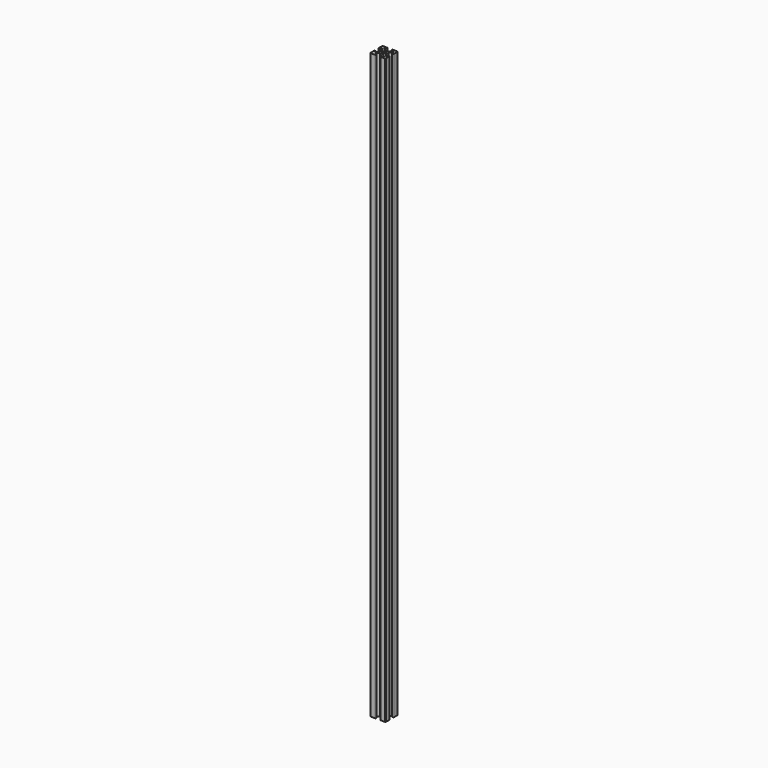
from build123d import *

# Parameters (mm, degrees)
F2_DEPTH = 760
F4_R     = 0.5
F5_R     = 1
F6_COUNT = 4


with BuildPart() as f2:
    # F1 (on Top) → F2 (new body)
    with BuildSketch(Plane.XY):
        with BuildLine():
            Line((3.0000000262, 10), (3.0000000262, 8))
            Line((3.0000000262, 8), (6.0000000262, 8))
            Line((6.0000000262, 8), (6.0000000262, 7.6925075952))
            Line((6.0000000262, 7.6925075952), (2.290812958, 4.0206899498))
            Line((2.290812958, 4.0206899498), (0.2126651618, 4))
            Line((0.2126651618, 4), (-0.0373348382, 3.75))
            Line((-0.0373348382, 3.75), (-0.0209097774, 2.1002278027))
            ThreePointArc((-0.0209097774, 2.1002278027), (1.4776309645, 1.4925138011), (2.1, 0))
            Line((2.1, 0), (3.7501858474, 0))
            Line((3.7501858474, 0), (4.0001858474, 0.25))
            Line((4.0001858474, 0.25), (3.9833205532, 2.3281823546))
            Line((3.9833205532, 2.3281823546), (7.6925076214, 6))
            Line((7.6925076214, 6), (8.0000000262, 6))
            Line((8.0000000262, 6), (8.0000000262, 3))
            Line((8.0000000262, 3), (10.0000000262, 3))
            Line((10.0000000262, 3), (10.0000000262, 10))
            Line((10.0000000262, 10), (3.0000000262, 10))
        make_face()
    extrude(amount=F2_DEPTH)

    # F4
    f4_edges = [f2.edges().sort_by_distance(p)[0] for p in [
        (3, 10, 380),
        (10, 3, 380),
        (8, 3, 380),
        (3, 8, 380),
    ]]
    fillet(f4_edges, radius=F4_R)

    # F5
    f5_edges = [f2.edges().sort_by_distance(p)[0] for p in [
        (10, 10, 380),
    ]]
    fillet(f5_edges, radius=F5_R)

    # F6: F2 ×4 about axis
    f6_axis = Axis((0, 0, 380), (0, 0, 1))


with BuildPart() as f2_1:
    add(f2.part)
    for i in range(1, F6_COUNT):
        add(f2.part.rotate(f6_axis, i * 360 / F6_COUNT))


solid = f2_1.part
